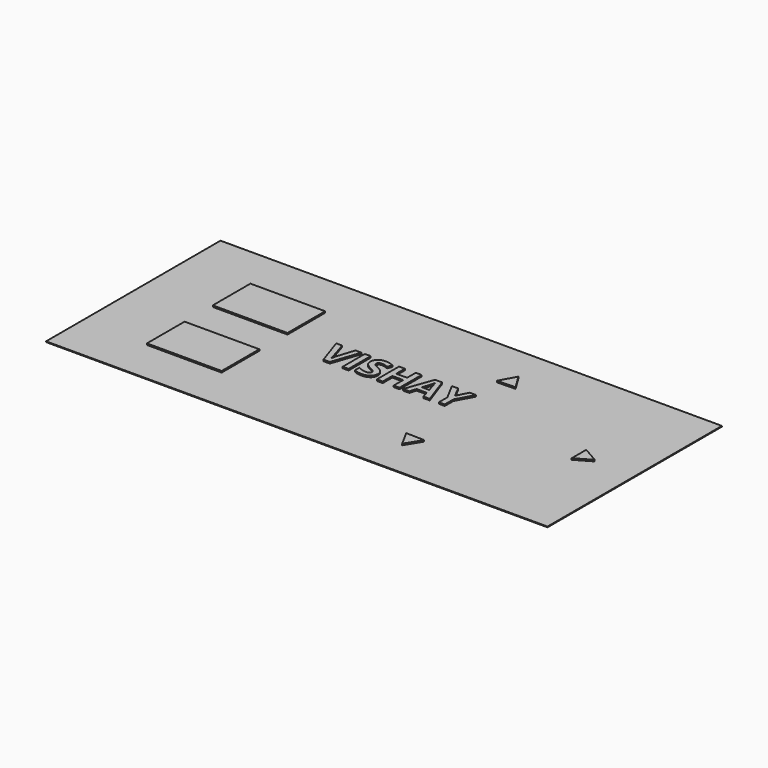
from build123d import *

# Parameters (mm, degrees)
F0_W         = 6.9
F0_H         = 3
F1_DEPTH     = 0.01
F2_W         = 1.0281072708
F2_H         = 0.6472328721
F2_TEXT_SIZE = 0.5328998466
F3_DEPTH     = 0.02


# Not quite as in the source:
# - Text() gives the source's letters only with a copy of the font that has no kerning and outlines rounded to 1/6400 em; it was checked with that copy


with BuildPart() as f1:
    # F0 (on Top) → F1 (new body)
    with BuildSketch(Plane.XY):
        Rectangle(F0_W, F0_H)
    extrude(amount=F1_DEPTH)

    # F2 (on face) → F3 (join)
    with BuildSketch(Plane.XY.offset(0.01)):
        Polygon((1.1806523823, 0.7868569612), (1.05, 1), (0.9307389049, 0.7802801985), align=None)
        Polygon((1.1806523823, -0.7868569612), (0.9307389049, -0.7802801985), (1.05, -1), align=None)
        with Locations((-2.0359463646, 0.566383564)):
            Rectangle(F2_W, F2_H)
        with Locations((-2.0359463646, -0.566383564)):
            Rectangle(F2_W, F2_H)
        Polygon((2.6834936491, -0.125), (2.9, 0), (2.6834936491, 0.125), align=None)
        with Locations((-0.9621340199, 0)):
            Text('VISHAY', F2_TEXT_SIZE, font='Open Sans', font_style=FontStyle.BOLD, text_align=(TextAlign.LEFT, TextAlign.BOTTOM))
    extrude(amount=F3_DEPTH)


solid = f1.part
